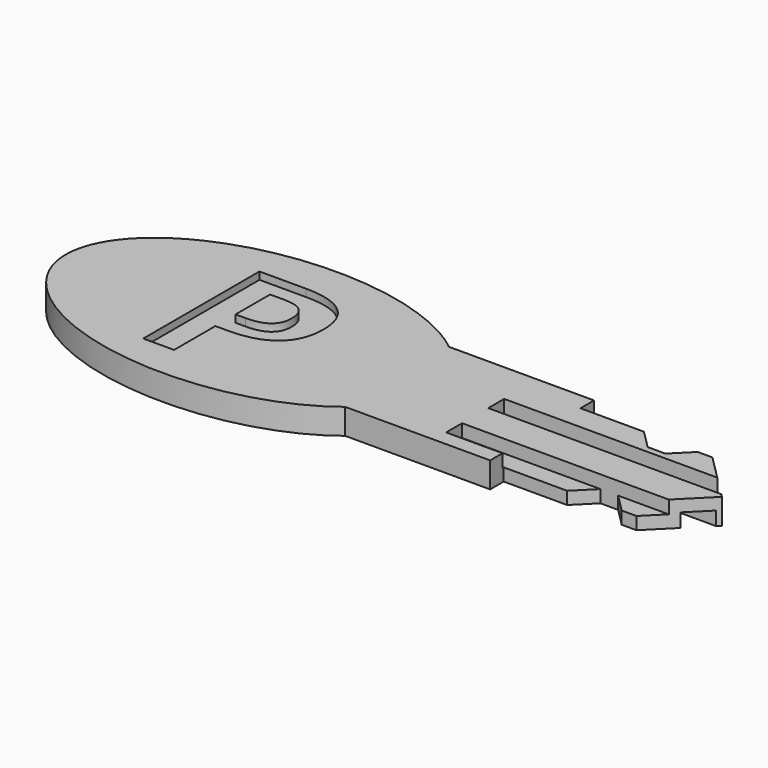
from build123d import *

# Parameters (mm, degrees)
F0_W         = 22
F0_H         = 8.8
F1_DEPTH     = 1.73
F2_W         = 1.35
F2_H         = 0.88
F2_H_2       = 0.93
F3_DEPTH     = 16
F4_W         = 12.18
F4_H         = 1.05
F5_DEPTH     = 1.73
F7_DEPTH     = 1.73
F8_TEXT_SIZE = 13.7823171259
F9_DEPTH     = 0.5


# Not quite as in the source:
# - Text() gives the source's letters only with a copy of the font that has no kerning and outlines rounded to 1/6400 em; it was checked with that copy


with BuildPart() as f1:
    # F0 (on Top) → F1 (new body)
    with BuildSketch(Plane.XY):
        with Locations((0.7483828813, 0)):
            Rectangle(F0_W, F0_H)
    extrude(amount=F1_DEPTH)

    # F2 (on face) → F3 (cut)
    with BuildSketch(Plane.YZ.offset(11.7483828813)):
        with Locations((-2.675, 1.29)):
            Rectangle(F2_W, F2_H)
        with Locations((-0.8916666667, 0.465)):
            Rectangle(F2_W, F2_H_2)
        with Locations((0.8916666667, 1.265)):
            Rectangle(F2_W, F2_H_2)
        with Locations((2.675, 0.44)):
            Rectangle(F2_W, F2_H)
    extrude(amount=-F3_DEPTH, mode=Mode.SUBTRACT)

    # F4 (on face) → F5 (cut, through all)
    with BuildSketch(Plane.XY.offset(1.73)):
        Polygon((11.7483828813, 4.4), (-0.4316171187, 4.4), (-0.4316171187, 3.25), (2.4791492486, 3.25), (3.8683828813, 3.25), (5.1192207954, 1.9991620859), (6.3192207954, 1.9991620859), (7.5342207954, 3.2141620859), (8.5342207954, 3.2141620859), (10.1817162146, 1.5666666667), (11.7483828813, 1.5666666667), align=None)
        with Locations((5.6583828813, -3.875)):
            Rectangle(F4_W, F4_H)
        Polygon((-0.4316171187, -3.25), (-0.4316171187, -3.35), (11.7483828813, -3.35), (11.7483828813, -2), (9.7483828813, -2), (8.5342207954, -3.2141620859), (7.5342207954, -3.2141620859), (6.3200587096, -2), (5.1183828813, -2), (3.8683828813, -3.25), (2.4791492486, -3.25), align=None)
        Polygon((11.7483828813, -2), (11.7483828813, 0), (9.7483828813, -2), align=None)
        Polygon((11.7483828813, 0.2166666667), (11.7483828813, 1.5666666667), (10.1817162146, 1.5666666667), (11.5317162146, 0.2166666667), align=None)
        Polygon((11.7483828813, 0), (11.7483828813, 0.2166666667), (11.5317162146, 0.2166666667), align=None)
    extrude(amount=-F5_DEPTH, mode=Mode.SUBTRACT)

    # F6 (on face) → F7 (join, through all)
    with BuildSketch(Plane(origin=(0, 0, 0), x_dir=(1, 0, 0), z_dir=(0, 0, -1))):
        with BuildLine():
            add(Edge.make_bspline(
                [(-7.811850141, 0), (-7.811850141, 12.8127456016), (-26.4715006076, 6.4063728008), (-45.1311510741, 0), (-26.4715006076, -6.4063728008), (-7.811850141, -12.8127456016), (-7.811850141, 0)],
                knots=[0, 0, 0, 2.0943951024, 2.0943951024, 4.1887902048, 4.1887902048, 6.2831853072, 6.2831853072, 6.2831853072], degree=2, weights=[1, 0.5, 1, 0.5, 1, 0.5, 1]))
        make_face()
    extrude(amount=-F7_DEPTH)

    # F8 (on face) → F9 (cut)
    with BuildSketch(Plane.XY.offset(1.73)):
        with Locations((-24.7157957753, -4.9616341653)):
            Text('P', F8_TEXT_SIZE, font='Open Sans', font_style=FontStyle.BOLD, text_align=(TextAlign.LEFT, TextAlign.BOTTOM))
    extrude(amount=-F9_DEPTH, mode=Mode.SUBTRACT)


solid = f1.part
